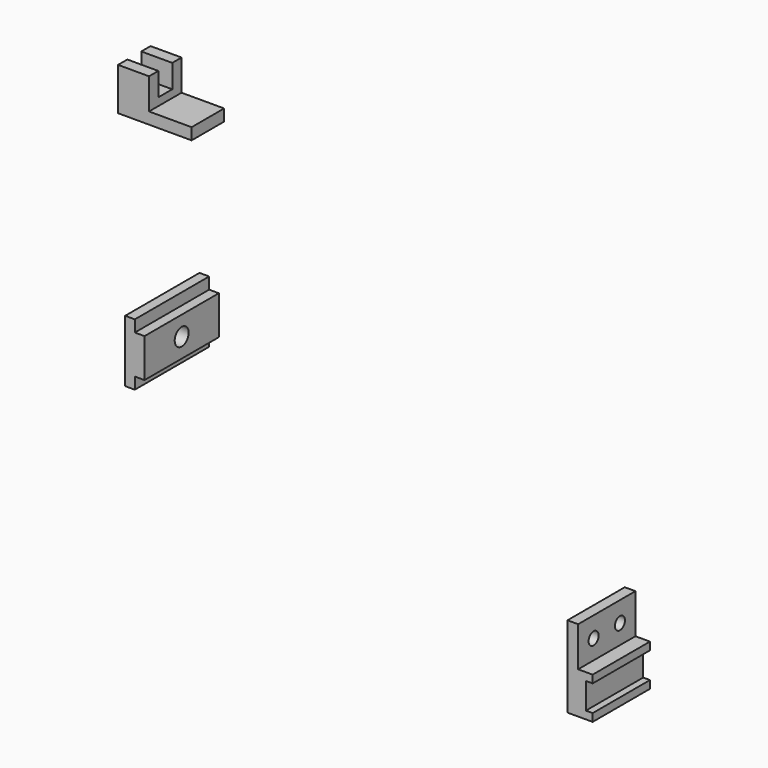
from build123d import *

# Parameters (mm, degrees)
F1_DEPTH  = 152.4
F2_R      = 14.2875
F3_DEPTH  = 25.4
F4_DEPTH  = 6.351
F6_DEPTH  = 117.475
F8_R      = 10.31875
F9_DEPTH  = 837.0034227142
F13_DEPTH = 66.675
F15_W     = 25.4
F15_H     = 19.05
F16_DEPTH = 25.4
F17_DEPTH = 25.4
F18_DEPTH = 67.0933896
F19_W     = 25.4
F19_H     = 25.4
F20_DEPTH = 19.05
F21_DEPTH = 25.4


# Not quite as in the source:
# - the program builds the solid bodies; features that only make, move or delete a surface that nothing else refers to are left out


with BuildPart() as f1:
    # F0 (on Front) → F1 (new body)
    with BuildSketch(Plane.XZ):
        Polygon((0, 48.9576303571), (-15.875, 48.9576303571), (-15.875, -52.6423696429), (0, -52.6423696429), (0, -33.5923696429), (15.875, -33.5923696429), (15.875, 29.9076303571), (0, 29.9076303571), align=None)
    extrude(amount=F1_DEPTH)

    # F2 (on face) → F3 (cut)
    with BuildSketch(Plane.YZ.offset(15.875)):
        with Locations((-76.2, -1.8423696429)):
            Circle(F2_R)
    extrude(amount=-F3_DEPTH, mode=Mode.SUBTRACT)

    # F4 (cut, through all): a face of the model
    f4_faces = [f1.faces().sort_by_distance(p)[0] for p in [
        (-9.525, -76.2, -1.8423696429),
    ]]
    extrude(f4_faces, amount=-F4_DEPTH, mode=Mode.SUBTRACT)


with BuildPart() as f6:
    # F5 (on face) → F6 (new body)
    with BuildSketch(Plane.XZ.offset(152.4)):
        Polygon((821.1274227142, -76.4874068737), (803.6649227142, -76.4874068737), (803.6649227142, -209.8374068737), (827.4774227142, -209.8374068737), (844.9399227142, -209.8374068737), (844.9399227142, -197.1374068737), (833.8274227142, -197.1374068737), (833.8274227142, -154.2749068737), (844.9399227142, -154.2749068737), (844.9399227142, -141.5749068737), (821.1274227142, -141.5749068737), align=None)
    extrude(amount=F6_DEPTH)

    # F8 (on face) → F9 (cut, through all)
    with BuildSketch(Plane.YZ.offset(821.1274227142)):
        with Locations((-184.15, -109.8249068737)):
            Circle(F8_R)
        with Locations((-238.125, -109.8249068737)):
            Circle(F8_R)
    extrude(amount=-F9_DEPTH, mode=Mode.SUBTRACT)


with BuildPart() as f13:
    # F12 (on face) → F13 (new body)
    with BuildSketch(Plane.XZ.offset(152.4)):
        Polygon((51.2173896, 426.5687932044), (25.8173896, 426.5687932044), (25.8173896, 382.1187932044), (146.4673896, 382.1187932044), (146.4673896, 401.1687932044), (51.2173896, 401.1687932044), align=None)
    extrude(amount=F13_DEPTH)

    # F15 (on face) → F16 (join)
    with BuildSketch(Plane.XY.offset(426.5687932044)):
        with Locations((38.5173896, -209.55)):
            Rectangle(F15_W, F15_H)
        with Locations((38.5173896, -161.925)):
            Rectangle(F15_W, F15_H)
    extrude(amount=F16_DEPTH)

    # F14 (on face) → F17 (join)
    with BuildSketch(Plane.YZ.offset(51.2173896)):
        Polygon((-200.025, 413.8687932044), (-200.025, 426.5687932044), (-219.075, 426.5687932044), (-219.075, 401.1687932044), (-152.4, 401.1687932044), (-152.4, 426.5687932044), (-171.45, 426.5687932044), (-171.45, 413.8687932044), align=None)
    extrude(amount=F17_DEPTH)

    # F18 (cut, through all): a face of the model
    f18_faces = [f13.faces().sort_by_distance(p)[0] for p in [
        (51.2173896, -185.7375, 420.2187932044),
    ]]
    extrude(f18_faces, amount=-F18_DEPTH, mode=Mode.SUBTRACT)

    # F19 (on face) → F20 (join)
    with BuildSketch(Plane.XZ.offset(219.075)):
        with Locations((63.9173896, 439.2687932044)):
            Rectangle(F19_W, F19_H)
    extrude(amount=-F20_DEPTH)

    # F21 (add): a face of the model
    f21_faces = [f13.faces().sort_by_distance(p)[0] for p in [
        (51.2173896, -161.925, 439.2687932044),
    ]]
    extrude(f21_faces, amount=F21_DEPTH)


solid = Compound([f1.part, f6.part, f13.part])
